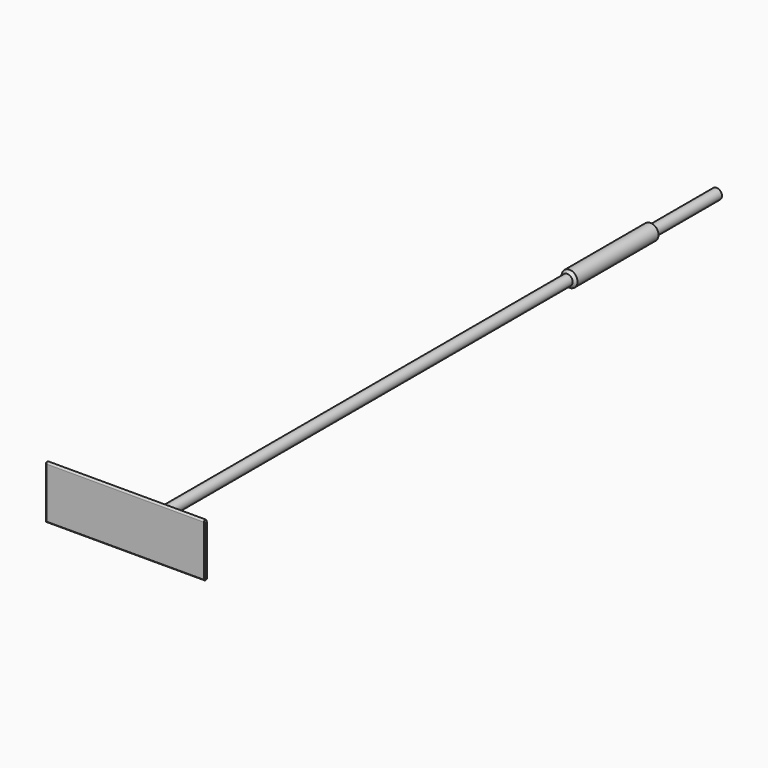
from build123d import *

# Parameters (mm, degrees)
F0_R     = 10
F1_DEPTH = 1406
F2_R     = 7.5
F3_DEPTH = 1800
F6_DEPTH = 300
F8_R     = 15
F9_DEPTH = 200
F10_SIZE = 4.99999
F11_SIZE = 1
F12_SIZE = 2


# Not quite as in the source:
# - a fillet or chamfer is up to 0.001 mm smaller than in the source, because OpenCascade refuses the exact size
# - a feature names something its author has since deleted; it is built from what else it names


with BuildPart() as f1:
    # F0 (on Front) → F1 (new body)
    with BuildSketch(Plane.XZ):
        Circle(F0_R)
    extrude(amount=-F1_DEPTH)

    # F2 (on Front) → F3 (cut)
    with BuildSketch(Plane.XZ):
        Circle(F2_R)
    extrude(amount=-F3_DEPTH, mode=Mode.SUBTRACT)

    # F5 (on offset) → F6 (join)
    with BuildSketch(Plane.YZ.offset(165)):
        with BuildLine():
            Line((0, 82), (0, -15))
            Line((0, -15), (6, -15))
            Line((6, -15), (6, 82))
            ThreePointArc((6, 82), (3, 85), (0, 82))
        make_face()
    extrude(amount=-F6_DEPTH)

    # F8 (on offset) → F9 (join)
    with BuildSketch(Plane.XZ.offset(-1256)):
        Circle(F8_R)
    extrude(amount=F9_DEPTH)

    # F10 (size 5 in the source; OpenCascade refuses exactly that, so slightly less here)
    f10_edges = [f1.edges().sort_by_distance(p)[0] for p in [
        (15, 1156, 0),
        (-15, 1256, 0),
        (-15, 1056, 0),
    ]]
    chamfer(f10_edges, length=F10_SIZE)

    # F11
    f11_edges = [f1.edges().sort_by_distance(p)[0] for p in [
        (-10, 6, 0),
    ]]
    chamfer(f11_edges, length=F11_SIZE)

    # F12
    f12_edges = [f1.edges().sort_by_distance(p)[0] for p in [
        (165, 0, 33.5),
        (165, 3, -15),
        (165, 6, 33.5),
        (165, 3, 85),
        (15, 0, -15),
        (15, 6, -15),
        (15, 6, 82),
        (-135, 6, 33.5),
        (-135, 0, 33.5),
        (15, 0, 82),
        (-135, 3, 85),
    ]]
    chamfer(f12_edges, length=F12_SIZE)


solid = f1.part
